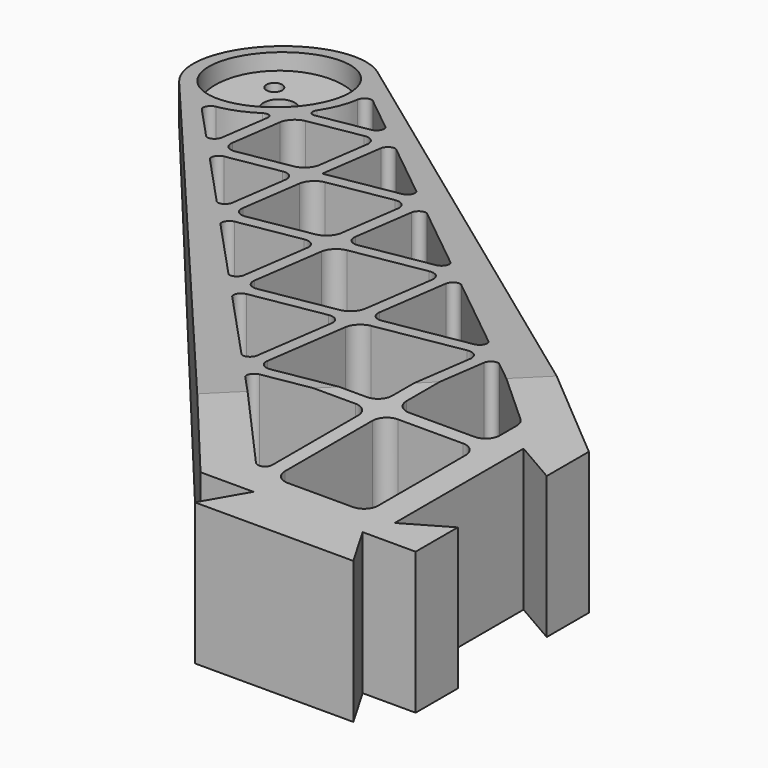
from build123d import *

# Parameters (mm, degrees)
F1_DEPTH       = 31.75
F2_R           = 14.325
F3_DEPTH       = 28.575
F5_DEPTH       = 31.75
F7_DEPTH       = 31.751
F9_DEPTH       = 31.751
F10_W          = 27.8922222136
F10_H          = 28.1136979927
F10_W_2        = 22.0070765571
F10_H_2        = 22.18663187
F10_W_3        = 19.4776418147
F10_H_3        = 19.6770581923
F10_W_4        = 24.7722447466
F10_H_4        = 25.0182185186
F11_DEPTH      = 31.75
F12_R          = 1.524
F13_R          = 1.524
F14_R          = 3.175
F16_DEPTH      = 31.75
F20_DEPTH      = 131.1291589461
F20_DEPTH_BACK = 124.3230200021
F21_R          = 3.5
F21_R_2        = 1.75
F22_DEPTH      = 31.751


# Not quite as in the source:
# - a feature names something its author has since deleted; it is built from what else it names


with BuildPart() as f1:
    # F0 (on Top) → F1 (new body)
    with BuildSketch(Plane.XY):
        with BuildLine():
            ThreePointArc((-171.2164076011, 147.819121873), (-151.8134645157, 142.5585953186), (-140.2663976585, 159.0149797027))
            ThreePointArc((-140.2663976585, 159.0149797027), (-141.8914670948, 166.3795285416), (-146.4648638984, 172.3763170112))
            ThreePointArc((-146.4648638984, 172.3763170112), (-170.0918974756, 171.438024992), (-171.2164076011, 147.819121873))
        make_face()
        with BuildLine():
            ThreePointArc((-146.4648638984, 172.3763170112), (-141.8914670948, 166.3795285416), (-140.2663976585, 159.0149797027))
            ThreePointArc((-140.2663976585, 159.0149797027), (-151.8134645157, 142.5585953186), (-171.2164076011, 147.819121873))
            Line((-171.2164076011, 147.819121873), (-48.1710061431, 0))
            Line((-48.1710061431, 0), (0, 0))
            Line((0, 0), (0, 48.4906934548))
            Line((0, 48.4906934548), (-146.4648638984, 172.3763170112))
        make_face()
    extrude(amount=F1_DEPTH)

    # F2 (on face) → F3 (cut)
    with BuildSketch(Plane.XY.offset(31.75)):
        with Locations((-157.7663976585, 159.0149797027)):
            Circle(F2_R)
    extrude(amount=-F3_DEPTH, mode=Mode.SUBTRACT)

    # F4 (on face) → F5 (join)
    with BuildSketch(Plane.XY.offset(31.75)):
        Polygon((-11.849261314, 0), (-36.3217448291, 0), (-41.8210061431, -9.525), (-6.35, -9.525), align=None)
    extrude(amount=-F5_DEPTH)

    # F6 (on face) → F7 (cut, through all)
    with BuildSketch(Plane.XY.offset(31.75)):
        Polygon((-9.652, 6.223), (0, 11.7955847982), (0, 36.6951086566), (-9.652, 42.2676934548), align=None)
    extrude(amount=-F7_DEPTH, mode=Mode.SUBTRACT)

    # F8 (on face) → F9 (cut, through all)
    with BuildSketch(Plane.XY.offset(31.75)):
        with BuildLine():
            Line((-16.002, 49.699371019), (-140.6956326235, 162.8671195132))
            ThreePointArc((-140.6956326235, 162.8671195132), (-140.3740374375, 160.9529698843), (-140.2663976585, 159.0149797027))
            ThreePointArc((-140.2663976585, 159.0149797027), (-146.8924666341, 145.3033924833), (-161.7529832673, 141.9751107131))
            Line((-161.7529832673, 141.9751107131), (-40.600106963, 6.35))
            Line((-40.600106963, 6.35), (-16.002, 6.35))
            Line((-16.002, 6.35), (-16.002, 49.699371019))
        make_face()
    extrude(amount=-F9_DEPTH, mode=Mode.SUBTRACT)

    # F10 (on face) → F11 (join, through all)
    with BuildSketch(Plane.XY.offset(31.75)):
        with BuildLine():
            ThreePointArc((-144.01445162, 148.1921344135), (-145.4358718483, 146.5969229609), (-147.0410978414, 145.1868220585))
            Line((-147.0410978414, 145.1868220585), (-147.0410978414, 125.5058270234))
            Line((-147.0410978414, 125.5058270234), (-144.0114513942, 122.1142762212))
            Line((-144.0114513942, 122.1142762212), (-124.3630560267, 122.1142762212))
            Line((-124.3630560267, 122.1142762212), (-124.3630560267, 100.1187951534))
            Line((-124.3630560267, 100.1187951534), (-121.3334095795, 96.7272443512))
            Line((-121.3334095795, 96.7272443512), (-99.1555794696, 96.7272443512))
            Line((-99.1555794696, 96.7272443512), (-99.1555794696, 71.9001766348))
            Line((-99.1555794696, 71.9001766348), (-96.1259330223, 68.5086258326))
            Line((-96.1259330223, 68.5086258326), (-71.182934723, 68.5086258326))
            Line((-71.182934723, 68.5086258326), (-71.182934723, 40.5860786421))
            Line((-71.182934723, 40.5860786421), (-68.1532882758, 37.1945278399))
            Line((-68.1532882758, 37.1945278399), (-40.0903125094, 37.1945278399))
            Line((-40.0903125094, 37.1945278399), (-40.0903125094, 6.35))
            Line((-40.0903125094, 6.35), (-36.8899125094, 6.35))
            Line((-36.8899125094, 6.35), (-36.8899125094, 37.1945278399))
            Line((-36.8899125094, 37.1945278399), (-16.002, 37.1945278399))
            Line((-16.002, 37.1945278399), (-16.002, 40.3949278399))
            Line((-16.002, 40.3949278399), (-36.8899125094, 40.3949278399))
            Line((-36.8899125094, 40.3949278399), (-36.8899125094, 68.6565381148))
            Line((-36.8899125094, 68.6565381148), (-40.2532893295, 71.7090258326))
            Line((-40.2532893295, 71.7090258326), (-67.982534723, 71.7090258326))
            Line((-67.982534723, 71.7090258326), (-67.982534723, 96.8751566334))
            Line((-67.982534723, 96.8751566334), (-71.3459115431, 99.9276443512))
            Line((-71.3459115431, 99.9276443512), (-95.9551794696, 99.9276443512))
            Line((-95.9551794696, 99.9276443512), (-95.9551794696, 122.2621885034))
            Line((-95.9551794696, 122.2621885034), (-99.3185562896, 125.3146762212))
            Line((-99.3185562896, 125.3146762212), (-121.1626560267, 125.3146762212))
            Line((-121.1626560267, 125.3146762212), (-121.1626560267, 145.1396466957))
            Line((-121.1626560267, 145.1396466957), (-124.5260328468, 148.1921344135))
            Line((-124.5260328468, 148.1921344135), (-144.01445162, 148.1921344135))
        make_face()
        with Locations((-54.0364236162, 54.4517768362)):
            Rectangle(F10_W, F10_H, mode=Mode.SUBTRACT)
        with Locations((-110.1591177481, 111.0209602862)):
            Rectangle(F10_W_2, F10_H_2, mode=Mode.SUBTRACT)
        with Locations((-134.101876934, 135.1532053173)):
            Rectangle(F10_W_3, F10_H_3, mode=Mode.SUBTRACT)
        with Locations((-83.5690570963, 84.2181350919)):
            Rectangle(F10_W_4, F10_H_4, mode=Mode.SUBTRACT)
    extrude(amount=-F11_DEPTH)

    # F12
    f12_edges = [f1.edges().sort_by_distance(p)[0] for p in [
        (-147.041098, 145.186822, 15.875),
        (-161.752983, 141.975111, 15.875),
        (-147.041098, 125.505827, 15.875),
        (-140.695633, 162.86712, 15.875),
        (-144.014452, 148.192134, 15.875),
        (-124.526033, 148.192134, 15.875),
    ]]
    fillet(f12_edges, radius=F12_R)

    # F13
    f13_edges = [f1.edges().sort_by_distance(p)[0] for p in [
        (-124.363056, 100.118795, 15.875),
        (-144.011451, 122.114276, 15.875),
        (-121.33341, 96.727244, 15.875),
        (-99.155579, 71.900177, 15.875),
        (-71.182935, 40.586079, 15.875),
        (-96.125933, 68.508626, 15.875),
        (-95.955179, 122.262189, 15.875),
        (-121.162656, 145.139647, 15.875),
        (-67.982535, 96.875157, 15.875),
        (-99.318556, 125.314676, 15.875),
        (-71.345912, 99.927644, 15.875),
        (-40.253289, 71.709026, 15.875),
        (-68.153288, 37.194528, 15.875),
        (-36.889913, 68.656538, 15.875),
    ]]
    fillet(f13_edges, radius=F13_R)

    # F14
    f14_edges = [f1.edges().sort_by_distance(p)[0] for p in [
        (-40.090313, 40.394928, 15.875),
        (-67.982535, 40.394928, 15.875),
        (-67.982535, 68.508626, 15.875),
        (-40.090313, 68.508626, 15.875),
        (-40.090313, 37.194528, 15.875),
        (-16.002, 37.194528, 15.875),
        (-36.889913, 37.194528, 15.875),
        (-36.889913, 6.35, 15.875),
        (-16.002, 6.35, 15.875),
        (-71.182935, 68.508626, 15.875),
        (-71.182935, 71.709026, 15.875),
        (-67.982535, 71.709026, 15.875),
        (-95.955179, 71.709026, 15.875),
        (-95.955179, 96.727244, 15.875),
        (-71.182935, 96.727244, 15.875),
        (-99.155579, 96.727244, 15.875),
        (-99.155579, 122.114276, 15.875),
        (-124.363056, 122.114276, 15.875),
        (-124.363056, 144.991734, 15.875),
        (-95.955179, 99.927644, 15.875),
        (-121.162656, 99.927644, 15.875),
        (-143.840698, 125.314676, 15.875),
        (-99.155579, 99.927644, 15.875),
        (-124.363056, 125.314676, 15.875),
        (-121.162656, 122.114276, 15.875),
        (-143.840698, 144.991734, 15.875),
        (-36.889913, 40.394928, 15.875),
        (-16.002, 49.699371, 15.875),
        (-16.002, 40.394928, 15.875),
    ]]
    fillet(f14_edges, radius=F14_R)

    # F15 (on face) → F16 (join, through all)
    with BuildSketch(Plane.XY.offset(31.75)):
        with BuildLine():
            ThreePointArc((-40.0903125094, 9.9726537321), (-41.119997319, 8.4776111048), (-42.8839038824, 8.9066063266))
            Line((-42.8839038824, 8.9066063266), (-40.600106963, 6.35))
            Line((-40.600106963, 6.35), (-40.0903125094, 6.35))
            Line((-40.0903125094, 6.35), (-40.0903125094, 9.9726537321))
        make_face()
    extrude(amount=-F16_DEPTH)

    # F19 (on face) → F20 (cut, two sides)
    with BuildSketch(Plane(origin=(0, 0, 0), x_dir=(-0.7043142753, 0.7098883022, 0), z_dir=(0.7098883022, 0.7043142753, 0))) as f20_sk:
        Polygon((241.5, 6.35), (241.5, 31.75), (225.5252254981, 31.75), (63.5, 31.75), align=None)
    extrude(amount=-F20_DEPTH, mode=Mode.SUBTRACT)
    extrude(f20_sk.sketch, amount=F20_DEPTH_BACK, mode=Mode.SUBTRACT)

    # F21 (on face) → F22 (cut, through all)
    with BuildSketch(Plane(origin=(0, 0, 0), x_dir=(1, 0, 0), z_dir=(0, 0, -1))):
        with Locations((-157.7663976585, -159.0149797027)):
            Circle(F21_R)
        with Locations((-152.1318834564, -153.3358732848)):
            Circle(F21_R_2)
        with Locations((-163.4009118606, -164.6940861207)):
            Circle(F21_R_2)
        with Locations((-151.0224587872, -165.7059653177)):
            Circle(F21_R_2)
        with Locations((-164.5103365298, -152.3239940878)):
            Circle(F21_R_2)
    extrude(amount=-F22_DEPTH, mode=Mode.SUBTRACT)


solid = f1.part
